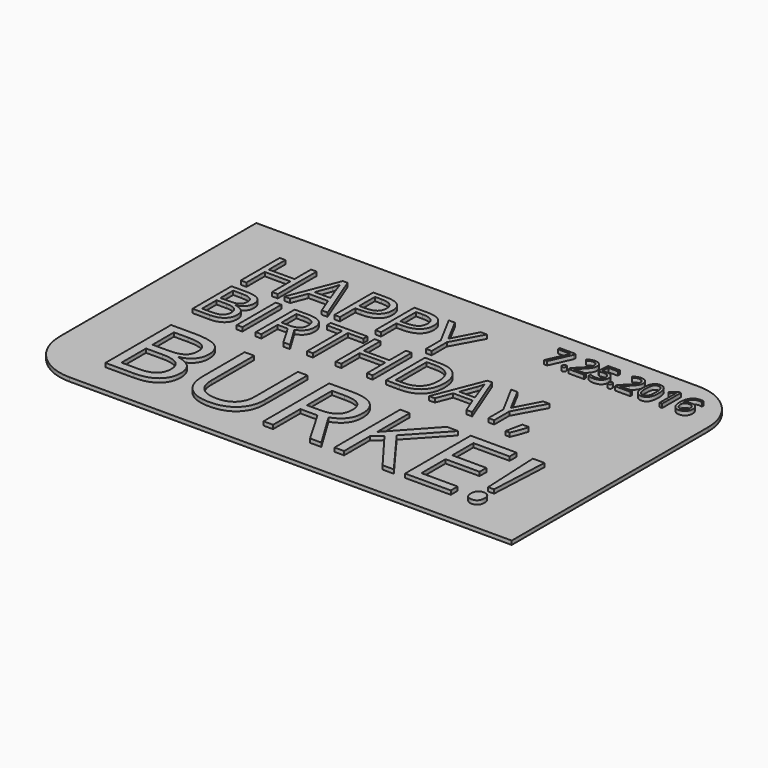
from build123d import *

# Parameters (mm, degrees)
F0_W           = 127
F0_H           = 76.2
F1_DEPTH       = 1
F2_TEXT_SIZE   = 17.6388888889
F2_TEXT_SIZE_2 = 29.7021743103
F2_TEXT_SIZE_3 = 8.4748905566
F3_DEPTH       = 1
F4_R           = 12.7


# Not quite as in the source:
# - Text() gives the source's letters only with a copy of the font that has no kerning and outlines rounded to 1/6400 em; it was checked with that copy


with BuildPart() as f1:
    # F0 (on Top) → F1 (new body)
    with BuildSketch(Plane.XY):
        with Locations((63.5, 38.1)):
            Rectangle(F0_W, F0_H)
    extrude(amount=F1_DEPTH)

    # F2 (on face) → F3 (join)
    with BuildSketch(Plane.XY.offset(1)):
        with Locations((12.7, 53.1472935933)):
            Text('HAPPY', F2_TEXT_SIZE, font='Open Sans', text_align=(TextAlign.LEFT, TextAlign.BOTTOM))
        with Locations((12.8252664581, 37.3973202288)):
            Text('BIRTHDAY,', F2_TEXT_SIZE, font='Open Sans', text_align=(TextAlign.LEFT, TextAlign.BOTTOM))
        with Locations((12.7, 7.9412086068)):
            Text('BURKE!', F2_TEXT_SIZE_2, font='Open Sans', text_align=(TextAlign.LEFT, TextAlign.BOTTOM))
        with Locations((82.822740078, 64.2365664244)):
            Text('7.25.2016', F2_TEXT_SIZE_3, font='Open Sans', text_align=(TextAlign.LEFT, TextAlign.BOTTOM))
    extrude(amount=F3_DEPTH)

    # F4
    f4_edges = [f1.edges().sort_by_distance(p)[0] for p in [
        (0, 0, 0.5),
        (127, 76.2, 0.5),
    ]]
    fillet(f4_edges, radius=F4_R)


solid = f1.part
